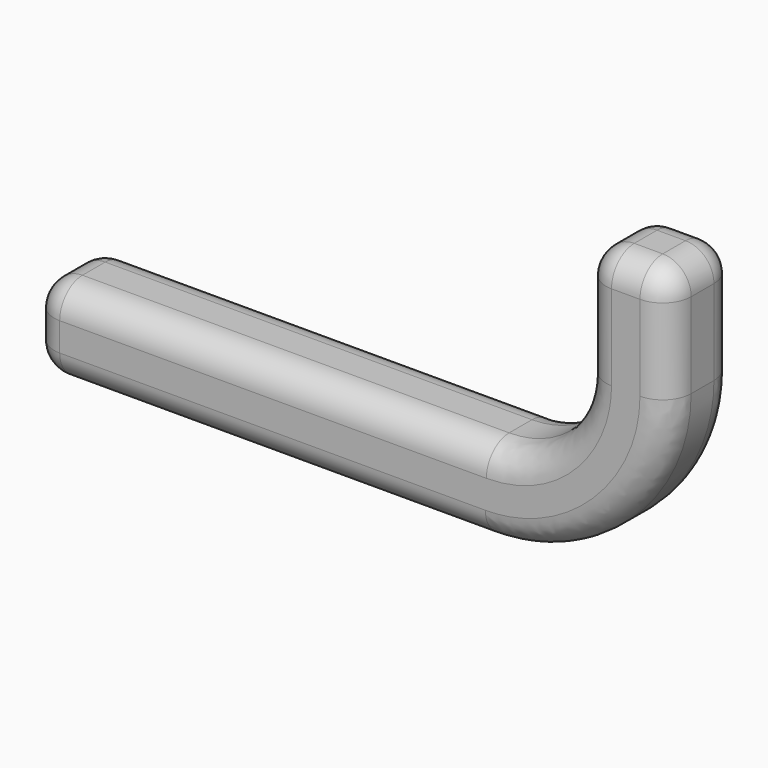
from build123d import *

# Parameters (mm, degrees)
F0_W     = 15
F0_H     = 20
F1_DEPTH = 15
F2_F1_R  = 5
F2_F2_R  = 5
F2_F3_R  = 5
F2_F4_R  = 5
F2_F5_R  = 5


# Not quite as in the source:
# - a feature of the source that left no trace in its solid (it failed there, or was rolled back) is left out
# - a feature names something its author has since deleted; it is built from what else it names


with BuildPart() as f1:
    # F0 (on Front) → F1 (new body)
    with BuildSketch(Plane.XZ):
        with BuildLine():
            add(Edge.make_bspline(
                [(80, 15), (90.0562568152, 15), (96.9973913685, 23.3758884073), (96.9973913685, 31.4775960116)],
                knots=[0, 0, 0, 0, 23.6732440459, 23.6732440459, 23.6732440459, 23.6732440459], degree=3))
            Line((80, 15), (79.8229584098, 0))
            add(Edge.make_bspline(
                [(111.9973913685, 31.4775960116), (111.9973913685, 15), (96.9973913685, 0), (79.8229584098, 0)],
                knots=[0, 0, 0, 0, 45.0114783904, 45.0114783904, 45.0114783904, 45.0114783904], degree=3))
            Line((111.9973913685, 31.4775960116), (96.9973913685, 31.4775960116))
        make_face()
        with Locations((104.4973913685, 41.4775960116)):
            Rectangle(F0_W, F0_H)
        Polygon((80, 15), (0, 15), (0, 0), (79.8229584098, 0), align=None)
    extrude(amount=F1_DEPTH)

    # F2: fillet of radius 5 on 20 edges, made by hand

    # F2_f1
    f2_f1_edges = [f1.edges().sort_by_distance(p)[0] for p in [
        (92.2697919899, 0, 20.2006576542),
        (96.9973913685, 0, 41.4775960116),
        (40, 0, 15),
    ]]
    fillet(f2_f1_edges, radius=F2_F1_R)

    # F2_f2
    f2_f2_edges = [f1.edges().sort_by_distance(p)[0] for p in [
        (92.2697919899, -15, 20.2006576542),
        (96.9973913685, -15, 41.4775960116),
        (40, -15, 15),
    ]]
    fillet(f2_f2_edges, radius=F2_F2_R)

    # F2_f3
    f2_f3_edges = [f1.edges().sort_by_distance(p)[0] for p in [
        (96.9973913685, -7.5, 51.4775960116),
    ]]
    fillet(f2_f3_edges, radius=F2_F3_R)

    # F2_f4
    f2_f4_edges = [f1.edges().sort_by_distance(p)[0] for p in [
        (111.9973913685, -7.5, 51.4775960116),
    ]]
    fillet(f2_f4_edges, radius=F2_F4_R)

    # F2_f5
    f2_f5_edges = [f1.edges().sort_by_distance(p)[0] for p in [
        (0, -7.5, 0),
    ]]
    fillet(f2_f5_edges, radius=F2_F5_R)


solid = f1.part
